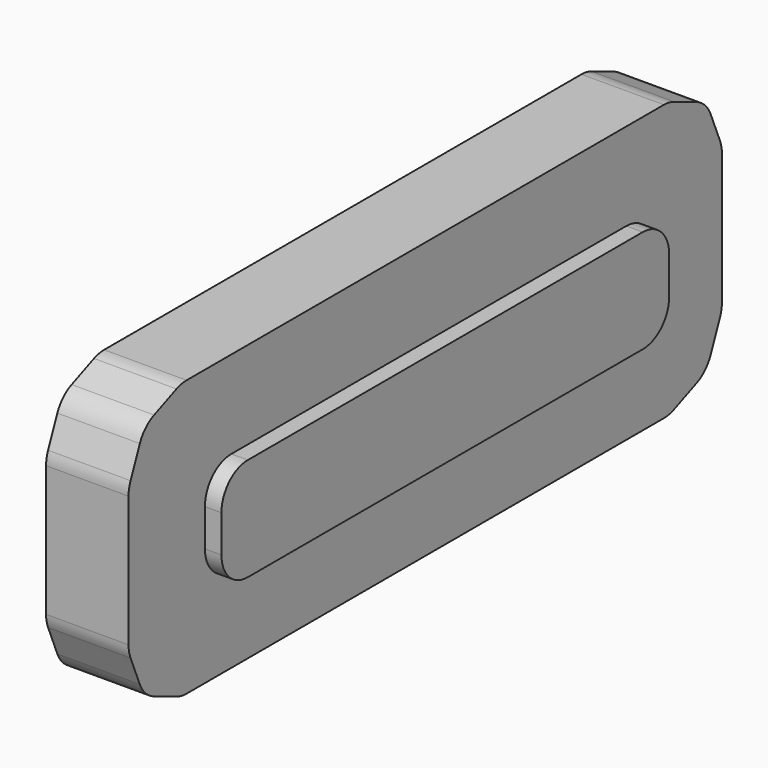
from build123d import *

# Parameters (mm, degrees)
F0_W        = 114.2217256129
F0_H        = 42.490478605
F1_DEPTH    = 12.7
F2_W        = 86.1872471869
F2_H        = 15.8843388781
F3_DEPTH    = 2.54
F4_R        = 5.08
F5_SIZE     = 5.08
F6_T1_DEPTH = 39.0415311919
F7_R        = 5.08


# Not quite as in the source:
# - a fillet or chamfer that OpenCascade refuses, or shapes differently, is made with other operations: its cross-section is extruded or revolved along the edge and cut away or added


with BuildPart() as f1:
    # F0 (on Right) → F1 (new body)
    with BuildSketch(Plane.YZ):
        with Locations((10.7826646417, 2.6869159192)):
            Rectangle(F0_W, F0_H)
    extrude(amount=F1_DEPTH)

    # F2 (on face) → F3 (join)
    with BuildSketch(Plane.YZ.offset(12.7)):
        with Locations((11.4720221609, 2.5003128685)):
            Rectangle(F2_W, F2_H)
    extrude(amount=F3_DEPTH)

    # F4
    f4_edges = [f1.edges().sort_by_distance(p)[0] for p in [
        (13.97, -31.621601, 10.442482),
        (13.97, -31.621601, -5.441857),
        (13.97, 54.565646, 10.442482),
        (13.97, 54.565646, -5.441857),
    ]]
    fillet(f4_edges, radius=F4_R)

    # F5
    f5_edges = [f1.edges().sort_by_distance(p)[0] for p in [
        (6.35, 67.893527, 23.932155),
        (6.35, 67.893527, -18.558323),
        (6.35, -46.328198, -18.558323),
        (6.35, -46.328198, 23.932155),
    ]]
    chamfer(f5_edges, length=F5_SIZE)

    # F6: chamfer of 5.08 on 8 edges, made by hand

    # F6_s2 → F6_t1 (cut)
    with BuildSketch(Plane.YZ.offset(-13.170765596)):
        Polygon((-42.7360957163, 22.4442576701), (-46.3281981647, 13.7721552217), (-46.3281981647, 18.8521552217), align=None)
        Polygon((-36.1681981647, 23.9321552217), (-44.8403006131, 20.3400527733), (-41.2481981647, 23.9321552217), align=None)
        Polygon((57.7335274482, 23.9321552217), (66.4056298966, 20.3400527733), (62.8135274482, 23.9321552217), align=None)
        Polygon((64.3014249997, 22.4442576701), (67.8935274482, 13.7721552217), (67.8935274482, 18.8521552217), align=None)
        Polygon((67.8935274482, -8.3983233833), (64.3014249997, -17.0704258318), (67.8935274482, -13.4783233833), align=None)
        Polygon((66.4056298966, -14.9662209349), (57.7335274482, -18.5583233833), (62.8135274482, -18.5583233833), align=None)
        Polygon((-46.3281981647, -8.3983233833), (-42.7360957163, -17.0704258318), (-46.3281981647, -13.4783233833), align=None)
        Polygon((-44.8403006131, -14.9662209349), (-36.1681981647, -18.5583233833), (-41.2481981647, -18.5583233833), align=None)
    extrude(amount=F6_T1_DEPTH, mode=Mode.SUBTRACT)

    # F7
    f7_edges = [f1.edges().sort_by_distance(p)[0] for p in [
        (6.35, -43.352403, -15.582528),
        (6.35, -36.168198, -18.558323),
        (6.35, -46.328198, -8.398323),
        (6.35, -43.352403, 20.95636),
        (6.35, -46.328198, 13.772155),
        (6.35, -36.168198, 23.932155),
        (6.35, 57.733527, 23.932155),
        (6.35, 64.917732, 20.95636),
        (6.35, 67.893527, 13.772155),
        (6.35, 67.893527, -8.398323),
        (6.35, 64.917732, -15.582528),
        (6.35, 57.733527, -18.558323),
    ]]
    fillet(f7_edges, radius=F7_R)


solid = f1.part
